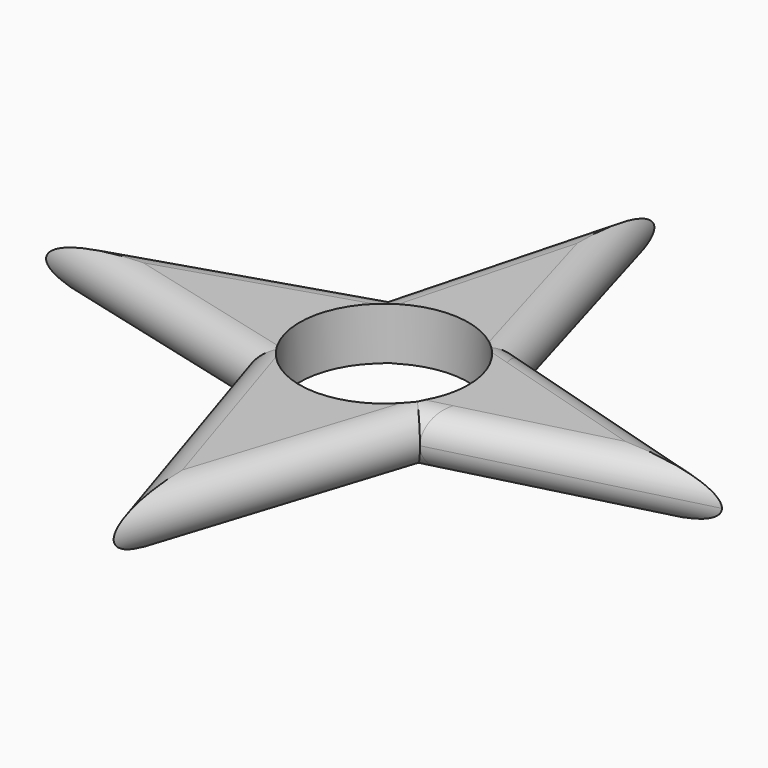
from build123d import *

# Parameters (mm, degrees)
F0_R         = 11.25
F1_DEPTH     = 7
F2_T4_DEPTH  = 53.5102509631
F2_T9_DEPTH  = 52.2381371755
F2_T14_DEPTH = 55.3419579342
F2_T19_DEPTH = 51.9229754131
F2_T24_DEPTH = 55.7195375849
F2_T29_DEPTH = 55.7195375849
F2_T34_DEPTH = 51.9229754131
F2_T39_DEPTH = 53.9484048993
F2_T45_DEPTH = 53.9484048993
F2_T49_DEPTH = 53.5102509631
F2_T56_DEPTH = 52.2381371755
F2_T60_DEPTH = 55.3419579342
F2_T67_DEPTH = 55.7195375849
F2_T71_DEPTH = 51.9229754131
F2_T78_DEPTH = 55.7195375849
F2_T82_DEPTH = 51.9229754131
F3_T4_DEPTH  = 53.5102509631
F3_T9_DEPTH  = 53.9484048993
F3_T14_DEPTH = 51.9229754131
F3_T19_DEPTH = 55.7195375849
F3_T24_DEPTH = 55.7195375849
F3_T29_DEPTH = 51.9229754131
F3_T34_DEPTH = 55.3419579342
F3_T39_DEPTH = 52.2381371755
F3_T45_DEPTH = 53.5102509631
F3_T49_DEPTH = 53.9484048993
F3_T56_DEPTH = 51.9229754131
F3_T60_DEPTH = 55.7195375849
F3_T67_DEPTH = 55.7195375849
F3_T71_DEPTH = 51.9229754131
F3_T78_DEPTH = 55.3419579342
F3_T82_DEPTH = 52.2381371755


# Not quite as in the source:
# - a fillet or chamfer that OpenCascade refuses, or shapes differently, is made with other operations: its cross-section is extruded or revolved along the edge and cut away or added


with BuildPart() as f1:
    # F0 (on Top) → F1 (new body)
    with BuildSketch(Plane.XY):
        with BuildLine():
            ThreePointArc((11.6700973746, -8.6057438533), (13.7743677156, -4.5295467802), (14.5, 0))
            ThreePointArc((14.5, 0), (13.3480283218, 5.6639332553), (10.0751531144, 10.4279091731))
            ThreePointArc((10.0751531144, 10.4279091731), (0.7621030803, 14.4799585253), (-8.9248468856, 11.4279091731))
            ThreePointArc((-8.9248468856, 11.4279091731), (-14.3657490464, 1.9685665686), (-11.6700973746, -8.6057438533))
            ThreePointArc((-11.6700973746, -8.6057438533), (0, -14.5), (11.6700973746, -8.6057438533))
        make_face()
        Circle(F0_R, mode=Mode.SUBTRACT)
        with BuildLine():
            ThreePointArc((10.0751531144, 10.4279091731), (13.3480283218, 5.6639332553), (14.5, 0))
            ThreePointArc((14.5, 0), (13.7743677156, -4.5295467802), (11.6700973746, -8.6057438533))
            Line((11.6700973746, -8.6057438533), (45, 0))
            Line((45, 0), (10.0751531144, 10.4279091731))
        make_face()
        with BuildLine():
            ThreePointArc((-8.9248468856, 11.4279091731), (0.7621030803, 14.4799585253), (10.0751531144, 10.4279091731))
            Line((10.0751531144, 10.4279091731), (0, 45))
            Line((0, 45), (-8.9248468856, 11.4279091731))
        make_face()
        with BuildLine():
            Line((0, -45), (11.6700973746, -8.6057438533))
            ThreePointArc((11.6700973746, -8.6057438533), (0, -14.5), (-11.6700973746, -8.6057438533))
            Line((-11.6700973746, -8.6057438533), (0, -45))
        make_face()
        with BuildLine():
            ThreePointArc((-11.6700973746, -8.6057438533), (-14.3657490464, 1.9685665686), (-8.9248468856, 11.4279091731))
            Line((-8.9248468856, 11.4279091731), (-45, 0))
            Line((-45, 0), (-11.6700973746, -8.6057438533))
        make_face()
    extrude(amount=F1_DEPTH)

    # F2: fillet of radius 3.5 on 8 edges, made by hand


with BuildPart() as f2_tool2:
    # F2_s3 → F2_t4 (new body)
    with BuildSketch(Plane(origin=(0.4357492619, -1.4952391183, 0), x_dir=(0, 0, 1), z_dir=(-0.2797856956, 0.9600624795, 0))):
        with BuildLine():
            ThreePointArc((3.5, 12.5903563019), (5.9748737342, 11.5652300361), (7, 9.0903563019))
            Line((7, 9.0903563019), (7, 12.5903563019))
            Line((7, 12.5903563019), (3.5, 12.5903563019))
        make_face()
    extrude(amount=F2_T4_DEPTH)

    split(bisect_by=Plane(origin=(3.6834089544, 12.3363650004, 0), x_dir=(0, 0, 1), z_dir=(0.2861005633, 0.958199597, 0)), keep=Keep.TOP)


with BuildPart() as f1_1:
    add(f1.part)

    # F2_t1: cut F2_tool2
    add(f2_tool2.part, mode=Mode.SUBTRACT)


with BuildPart() as f2_tool7:
    # F2_s8 → F2_t9 (new body)
    with BuildSketch(Plane(origin=(13.4212581193, 50.4859861874, 0), x_dir=(0, 0, 1), z_dir=(-0.2569178318, -0.9664332505, 0))):
        with BuildLine():
            ThreePointArc((3.5, 11.5613024332), (5.9748737342, 10.5361761674), (7, 8.0613024332))
            Line((7, 8.0613024332), (7, 11.5613024332))
            Line((7, 11.5613024332), (3.5, 11.5613024332))
        make_face()
    extrude(amount=F2_T9_DEPTH)

    split(bisect_by=Plane(origin=(-4.1039199091, 12.9550853833, 0), x_dir=(0, 0, 1), z_dir=(-0.3019904306, 0.9533109565, 0)), keep=Keep.TOP)


with BuildPart() as f1_2:
    add(f1_1.part)

    # F2_t6: cut F2_tool7
    add(f2_tool7.part, mode=Mode.SUBTRACT)


with BuildPart() as f2_tool12:
    # F2_s13 → F2_t14 (new body)
    with BuildSketch(Plane(origin=(3.5205438929, 1.1152400579, 0), x_dir=(0, 0, 1), z_dir=(-0.9533109565, -0.3019904306, 0))):
        with BuildLine():
            ThreePointArc((3.5, 13.5895693791), (5.9748737342, 12.5644431133), (7, 10.0895693791))
            Line((7, 10.0895693791), (7, 13.5895693791))
            Line((7, 13.5895693791), (3.5, 13.5895693791))
        make_face()
    extrude(amount=F2_T14_DEPTH)

    split(bisect_by=Plane(origin=(-11.1732270906, 2.9703047545, 0), x_dir=(0, 0, 1), z_dir=(-0.9664332505, 0.2569178318, 0)), keep=Keep.TOP)


with BuildPart() as f1_3:
    add(f1_2.part)

    # F2_t11: cut F2_tool12
    add(f2_tool12.part, mode=Mode.SUBTRACT)


with BuildPart() as f2_tool17:
    # F2_s18 → F2_t19 (new body)
    with BuildSketch(Plane(origin=(-50.6596510698, 13.0802656612, 0), x_dir=(0, 0, 1), z_dir=(0.9682458366, -0.25, 0))):
        with BuildLine():
            ThreePointArc((3.5, 11.25), (5.9748737342, 10.2248737342), (7, 7.75))
            Line((7, 7.75), (7, 11.25))
            Line((7, 11.25), (3.5, 11.25))
        make_face()
    extrude(amount=F2_T19_DEPTH)

    split(bisect_by=Plane(origin=(-13.0842545446, -4.1955665749, 0), x_dir=(0, 0, 1), z_dir=(-0.9522421894, -0.3053437616, 0)), keep=Keep.TOP)


with BuildPart() as f1_4:
    add(f1_3.part)

    # F2_t16: cut F2_tool17
    add(f2_tool17.part, mode=Mode.SUBTRACT)


with BuildPart() as f2_tool22:
    # F2_s23 → F2_t24 (new body)
    with BuildSketch(Plane(origin=(-1.2576007444, 3.9219418787, 0), x_dir=(0, 0, 1), z_dir=(0.3053437616, -0.9522421894, 0))):
        with BuildLine():
            ThreePointArc((3.5, 13.7404692741), (5.9748737342, 12.7153430082), (7, 10.2404692741))
            Line((7, 10.2404692741), (7, 13.7404692741))
            Line((7, 13.7404692741), (3.5, 13.7404692741))
        make_face()
    extrude(amount=F2_T24_DEPTH)

    split(bisect_by=Plane(origin=(-2.8125, -10.8927656612, 0), x_dir=(0, 0, 1), z_dir=(-0.25, -0.9682458366, 0)), keep=Keep.TOP)


with BuildPart() as f1_5:
    add(f1_4.part)

    # F2_t21: cut F2_tool22
    add(f2_tool22.part, mode=Mode.SUBTRACT)


with BuildPart() as f2_tool27:
    # F2_s28 → F2_t29 (new body)
    with BuildSketch(Plane(origin=(-15.756012459, -49.1365525821, 0), x_dir=(0, 0, 1), z_dir=(0.3053437616, 0.9522421894, 0))):
        with BuildLine():
            ThreePointArc((3.5, 13.7404692741), (5.9748737342, 12.7153430082), (7, 10.2404692741))
            Line((7, 10.2404692741), (7, 13.7404692741))
            Line((7, 13.7404692741), (3.5, 13.7404692741))
        make_face()
    extrude(amount=F2_T29_DEPTH)

    split(bisect_by=Plane(origin=(2.8125, -10.8927656612, 0), x_dir=(0, 0, 1), z_dir=(0.25, -0.9682458366, 0)), keep=Keep.TOP)


with BuildPart() as f1_6:
    add(f1_5.part)

    # F2_t26: cut F2_tool27
    add(f2_tool27.part, mode=Mode.SUBTRACT)


with BuildPart() as f2_tool32:
    # F2_s33 → F2_t34 (new body)
    with BuildSketch(Plane(origin=(0.3854463047, 0.0995218079, 0), x_dir=(0, 0, 1), z_dir=(0.9682458366, 0.25, 0))):
        with BuildLine():
            ThreePointArc((3.5, 11.25), (5.9748737342, 10.2248737342), (7, 7.75))
            Line((7, 7.75), (7, 11.25))
            Line((7, 11.25), (3.5, 11.25))
        make_face()
    extrude(amount=F2_T34_DEPTH)

    split(bisect_by=Plane(origin=(13.0842545446, -4.1955665749, 0), x_dir=(0, 0, 1), z_dir=(0.9522421894, -0.3053437616, 0)), keep=Keep.TOP)


with BuildPart() as f1_7:
    add(f1_6.part)

    # F2_t31: cut F2_tool32
    add(f2_tool32.part, mode=Mode.SUBTRACT)


with BuildPart() as f2_tool37:
    # F2_s38 → F2_t39 (new body)
    with BuildSketch(Plane(origin=(49.7008375193, -14.8397449293, 0), x_dir=(0, 0, 1), z_dir=(-0.958199597, 0.2861005633, 0))):
        with BuildLine():
            ThreePointArc((3.5, 12.8745253485), (5.9748737342, 11.8493990826), (7, 9.3745253485))
            Line((7, 9.3745253485), (7, 12.8745253485))
            Line((7, 12.8745253485), (3.5, 12.8745253485))
        make_face()
    extrude(amount=F2_T39_DEPTH)

    split(bisect_by=Plane(origin=(12.087528689, 3.5226015958, 0), x_dir=(0, 0, 1), z_dir=(0.9600624795, 0.2797856956, 0)), keep=Keep.TOP)


with BuildPart() as f1_8:
    add(f1_7.part)

    # F2_t36: cut F2_tool37
    add(f2_tool37.part, mode=Mode.SUBTRACT)


with BuildPart() as f2_tool43:
    # F2_s44 → F2_t45 (new body)
    with BuildSketch(Plane(origin=(49.7008375193, -14.8397449293, 0), x_dir=(0, 0, 1), z_dir=(-0.958199597, 0.2861005633, 0))):
        with BuildLine():
            ThreePointArc((3.5, 12.8745253485), (5.9748737342, 11.8493990826), (7, 9.3745253485))
            Line((7, 9.3745253485), (7, 12.8745253485))
            Line((7, 12.8745253485), (3.5, 12.8745253485))
        make_face()
    extrude(amount=F2_T45_DEPTH)

    split(bisect_by=Plane(origin=(12.087528689, 3.5226015958, 0), x_dir=(0, 0, 1), z_dir=(-0.9600624795, -0.2797856956, 0)), keep=Keep.TOP)


with BuildPart() as f2_tool47:
    # F2_s48 → F2_t49 (new body)
    with BuildSketch(Plane(origin=(0.4357492619, -1.4952391183, 0), x_dir=(0, 0, 1), z_dir=(-0.2797856956, 0.9600624795, 0))):
        with BuildLine():
            ThreePointArc((3.5, 12.5903563019), (5.9748737342, 11.5652300361), (7, 9.0903563019))
            Line((7, 9.0903563019), (7, 12.5903563019))
            Line((7, 12.5903563019), (3.5, 12.5903563019))
        make_face()
    extrude(amount=F2_T49_DEPTH)

    split(bisect_by=Plane(origin=(3.6834089544, 12.3363650004, 0), x_dir=(0, 0, 1), z_dir=(-0.2861005633, -0.958199597, 0)), keep=Keep.TOP)


with BuildPart() as f2_tool43_1:
    add(f2_tool43.part)

    # F2_t51: intersect F2_tool47
    add(f2_tool47.part, mode=Mode.INTERSECT)


with BuildPart() as f1_9:
    add(f1_8.part)

    # F2_t41: cut F2_tool43
    add(f2_tool43_1.part, mode=Mode.SUBTRACT)


with BuildPart() as f2_tool54:
    # F2_s55 → F2_t56 (new body)
    with BuildSketch(Plane(origin=(13.4212581193, 50.4859861874, 0), x_dir=(0, 0, 1), z_dir=(-0.2569178318, -0.9664332505, 0))):
        with BuildLine():
            ThreePointArc((3.5, 11.5613024332), (5.9748737342, 10.5361761674), (7, 8.0613024332))
            Line((7, 8.0613024332), (7, 11.5613024332))
            Line((7, 11.5613024332), (3.5, 11.5613024332))
        make_face()
    extrude(amount=F2_T56_DEPTH)

    split(bisect_by=Plane(origin=(-4.1039199091, 12.9550853833, 0), x_dir=(0, 0, 1), z_dir=(0.3019904306, -0.9533109565, 0)), keep=Keep.TOP)


with BuildPart() as f2_tool58:
    # F2_s59 → F2_t60 (new body)
    with BuildSketch(Plane(origin=(3.5205438929, 1.1152400579, 0), x_dir=(0, 0, 1), z_dir=(-0.9533109565, -0.3019904306, 0))):
        with BuildLine():
            ThreePointArc((3.5, 13.5895693791), (5.9748737342, 12.5644431133), (7, 10.0895693791))
            Line((7, 10.0895693791), (7, 13.5895693791))
            Line((7, 13.5895693791), (3.5, 13.5895693791))
        make_face()
    extrude(amount=F2_T60_DEPTH)

    split(bisect_by=Plane(origin=(-11.1732270906, 2.9703047545, 0), x_dir=(0, 0, 1), z_dir=(0.9664332505, -0.2569178318, 0)), keep=Keep.TOP)


with BuildPart() as f2_tool54_1:
    add(f2_tool54.part)

    # F2_t62: intersect F2_tool58
    add(f2_tool58.part, mode=Mode.INTERSECT)


with BuildPart() as f1_10:
    add(f1_9.part)

    # F2_t52: cut F2_tool54
    add(f2_tool54_1.part, mode=Mode.SUBTRACT)


with BuildPart() as f2_tool65:
    # F2_s66 → F2_t67 (new body)
    with BuildSketch(Plane(origin=(-1.2576007444, 3.9219418787, 0), x_dir=(0, 0, 1), z_dir=(0.3053437616, -0.9522421894, 0))):
        with BuildLine():
            ThreePointArc((3.5, 13.7404692741), (5.9748737342, 12.7153430082), (7, 10.2404692741))
            Line((7, 10.2404692741), (7, 13.7404692741))
            Line((7, 13.7404692741), (3.5, 13.7404692741))
        make_face()
    extrude(amount=F2_T67_DEPTH)

    split(bisect_by=Plane(origin=(-2.8125, -10.8927656612, 0), x_dir=(0, 0, 1), z_dir=(0.25, 0.9682458366, 0)), keep=Keep.TOP)


with BuildPart() as f2_tool69:
    # F2_s70 → F2_t71 (new body)
    with BuildSketch(Plane(origin=(-50.6596510698, 13.0802656612, 0), x_dir=(0, 0, 1), z_dir=(0.9682458366, -0.25, 0))):
        with BuildLine():
            ThreePointArc((3.5, 11.25), (5.9748737342, 10.2248737342), (7, 7.75))
            Line((7, 7.75), (7, 11.25))
            Line((7, 11.25), (3.5, 11.25))
        make_face()
    extrude(amount=F2_T71_DEPTH)

    split(bisect_by=Plane(origin=(-13.0842545446, -4.1955665749, 0), x_dir=(0, 0, 1), z_dir=(0.9522421894, 0.3053437616, 0)), keep=Keep.TOP)


with BuildPart() as f2_tool65_1:
    add(f2_tool65.part)

    # F2_t73: intersect F2_tool69
    add(f2_tool69.part, mode=Mode.INTERSECT)


with BuildPart() as f1_11:
    add(f1_10.part)

    # F2_t63: cut F2_tool65
    add(f2_tool65_1.part, mode=Mode.SUBTRACT)


with BuildPart() as f2_tool76:
    # F2_s77 → F2_t78 (new body)
    with BuildSketch(Plane(origin=(-15.756012459, -49.1365525821, 0), x_dir=(0, 0, 1), z_dir=(0.3053437616, 0.9522421894, 0))):
        with BuildLine():
            ThreePointArc((3.5, 13.7404692741), (5.9748737342, 12.7153430082), (7, 10.2404692741))
            Line((7, 10.2404692741), (7, 13.7404692741))
            Line((7, 13.7404692741), (3.5, 13.7404692741))
        make_face()
    extrude(amount=F2_T78_DEPTH)

    split(bisect_by=Plane(origin=(2.8125, -10.8927656612, 0), x_dir=(0, 0, 1), z_dir=(-0.25, 0.9682458366, 0)), keep=Keep.TOP)


with BuildPart() as f2_tool80:
    # F2_s81 → F2_t82 (new body)
    with BuildSketch(Plane(origin=(0.3854463047, 0.0995218079, 0), x_dir=(0, 0, 1), z_dir=(0.9682458366, 0.25, 0))):
        with BuildLine():
            ThreePointArc((3.5, 11.25), (5.9748737342, 10.2248737342), (7, 7.75))
            Line((7, 7.75), (7, 11.25))
            Line((7, 11.25), (3.5, 11.25))
        make_face()
    extrude(amount=F2_T82_DEPTH)

    split(bisect_by=Plane(origin=(13.0842545446, -4.1955665749, 0), x_dir=(0, 0, 1), z_dir=(-0.9522421894, 0.3053437616, 0)), keep=Keep.TOP)


with BuildPart() as f2_tool76_1:
    add(f2_tool76.part)

    # F2_t84: intersect F2_tool80
    add(f2_tool80.part, mode=Mode.INTERSECT)


with BuildPart() as f1_12:
    add(f1_11.part)

    # F2_t74: cut F2_tool76
    add(f2_tool76_1.part, mode=Mode.SUBTRACT)

    # F3: fillet of radius 3.5 on 8 edges, made by hand


with BuildPart() as f3_tool2:
    # F3_s3 → F3_t4 (new body)
    with BuildSketch(Plane(origin=(0.4357492619, -1.4952391183, 0), x_dir=(0, 0, 1), z_dir=(-0.2797856956, 0.9600624795, 0))):
        with BuildLine():
            ThreePointArc((3.5, 12.5903563019), (1.0251262658, 11.5652300361), (0, 9.0903563019))
            Line((0, 9.0903563019), (0, 12.5903563019))
            Line((0, 12.5903563019), (3.5, 12.5903563019))
        make_face()
    extrude(amount=F3_T4_DEPTH)

    split(bisect_by=Plane(origin=(3.6834089544, 12.3363650004, 0), x_dir=(0, 0, 1), z_dir=(0.2861005633, 0.958199597, 0)), keep=Keep.TOP)


with BuildPart() as f1_13:
    add(f1_12.part)

    # F3_t1: cut F3_tool2
    add(f3_tool2.part, mode=Mode.SUBTRACT)


with BuildPart() as f3_tool7:
    # F3_s8 → F3_t9 (new body)
    with BuildSketch(Plane(origin=(49.7008375193, -14.8397449293, 0), x_dir=(0, 0, 1), z_dir=(-0.958199597, 0.2861005633, 0))):
        with BuildLine():
            ThreePointArc((3.5, 12.8745253485), (1.0251262658, 11.8493990826), (0, 9.3745253485))
            Line((0, 9.3745253485), (0, 12.8745253485))
            Line((0, 12.8745253485), (3.5, 12.8745253485))
        make_face()
    extrude(amount=F3_T9_DEPTH)

    split(bisect_by=Plane(origin=(12.087528689, 3.5226015958, 0), x_dir=(0, 0, 1), z_dir=(0.9600624795, 0.2797856956, 0)), keep=Keep.TOP)


with BuildPart() as f1_14:
    add(f1_13.part)

    # F3_t6: cut F3_tool7
    add(f3_tool7.part, mode=Mode.SUBTRACT)


with BuildPart() as f3_tool12:
    # F3_s13 → F3_t14 (new body)
    with BuildSketch(Plane(origin=(0.3854463047, 0.0995218079, 0), x_dir=(0, 0, 1), z_dir=(0.9682458366, 0.25, 0))):
        with BuildLine():
            ThreePointArc((3.5, 11.25), (1.0251262658, 10.2248737342), (0, 7.75))
            Line((0, 7.75), (0, 11.25))
            Line((0, 11.25), (3.5, 11.25))
        make_face()
    extrude(amount=F3_T14_DEPTH)

    split(bisect_by=Plane(origin=(13.0842545446, -4.1955665749, 0), x_dir=(0, 0, 1), z_dir=(0.9522421894, -0.3053437616, 0)), keep=Keep.TOP)


with BuildPart() as f1_15:
    add(f1_14.part)

    # F3_t11: cut F3_tool12
    add(f3_tool12.part, mode=Mode.SUBTRACT)


with BuildPart() as f3_tool17:
    # F3_s18 → F3_t19 (new body)
    with BuildSketch(Plane(origin=(-15.756012459, -49.1365525821, 0), x_dir=(0, 0, 1), z_dir=(0.3053437616, 0.9522421894, 0))):
        with BuildLine():
            ThreePointArc((3.5, 13.7404692741), (1.0251262658, 12.7153430082), (0, 10.2404692741))
            Line((0, 10.2404692741), (0, 13.7404692741))
            Line((0, 13.7404692741), (3.5, 13.7404692741))
        make_face()
    extrude(amount=F3_T19_DEPTH)

    split(bisect_by=Plane(origin=(2.8125, -10.8927656612, 0), x_dir=(0, 0, 1), z_dir=(0.25, -0.9682458366, 0)), keep=Keep.TOP)


with BuildPart() as f1_16:
    add(f1_15.part)

    # F3_t16: cut F3_tool17
    add(f3_tool17.part, mode=Mode.SUBTRACT)


with BuildPart() as f3_tool22:
    # F3_s23 → F3_t24 (new body)
    with BuildSketch(Plane(origin=(-1.2576007444, 3.9219418787, 0), x_dir=(0, 0, 1), z_dir=(0.3053437616, -0.9522421894, 0))):
        with BuildLine():
            ThreePointArc((3.5, 13.7404692741), (1.0251262658, 12.7153430082), (0, 10.2404692741))
            Line((0, 10.2404692741), (0, 13.7404692741))
            Line((0, 13.7404692741), (3.5, 13.7404692741))
        make_face()
    extrude(amount=F3_T24_DEPTH)

    split(bisect_by=Plane(origin=(-2.8125, -10.8927656612, 0), x_dir=(0, 0, 1), z_dir=(-0.25, -0.9682458366, 0)), keep=Keep.TOP)


with BuildPart() as f1_17:
    add(f1_16.part)

    # F3_t21: cut F3_tool22
    add(f3_tool22.part, mode=Mode.SUBTRACT)


with BuildPart() as f3_tool27:
    # F3_s28 → F3_t29 (new body)
    with BuildSketch(Plane(origin=(-50.6596510698, 13.0802656612, 0), x_dir=(0, 0, 1), z_dir=(0.9682458366, -0.25, 0))):
        with BuildLine():
            ThreePointArc((3.5, 11.25), (1.0251262658, 10.2248737342), (0, 7.75))
            Line((0, 7.75), (0, 11.25))
            Line((0, 11.25), (3.5, 11.25))
        make_face()
    extrude(amount=F3_T29_DEPTH)

    split(bisect_by=Plane(origin=(-13.0842545446, -4.1955665749, 0), x_dir=(0, 0, 1), z_dir=(-0.9522421894, -0.3053437616, 0)), keep=Keep.TOP)


with BuildPart() as f1_18:
    add(f1_17.part)

    # F3_t26: cut F3_tool27
    add(f3_tool27.part, mode=Mode.SUBTRACT)


with BuildPart() as f3_tool32:
    # F3_s33 → F3_t34 (new body)
    with BuildSketch(Plane(origin=(3.5205438929, 1.1152400579, 0), x_dir=(0, 0, 1), z_dir=(-0.9533109565, -0.3019904306, 0))):
        with BuildLine():
            ThreePointArc((3.5, 13.5895693791), (1.0251262658, 12.5644431133), (0, 10.0895693791))
            Line((0, 10.0895693791), (0, 13.5895693791))
            Line((0, 13.5895693791), (3.5, 13.5895693791))
        make_face()
    extrude(amount=F3_T34_DEPTH)

    split(bisect_by=Plane(origin=(-11.1732270906, 2.9703047545, 0), x_dir=(0, 0, 1), z_dir=(-0.9664332505, 0.2569178318, 0)), keep=Keep.TOP)


with BuildPart() as f1_19:
    add(f1_18.part)

    # F3_t31: cut F3_tool32
    add(f3_tool32.part, mode=Mode.SUBTRACT)


with BuildPart() as f3_tool37:
    # F3_s38 → F3_t39 (new body)
    with BuildSketch(Plane(origin=(13.4212581193, 50.4859861874, 0), x_dir=(0, 0, 1), z_dir=(-0.2569178318, -0.9664332505, 0))):
        with BuildLine():
            ThreePointArc((3.5, 11.5613024332), (1.0251262658, 10.5361761674), (0, 8.0613024332))
            Line((0, 8.0613024332), (0, 11.5613024332))
            Line((0, 11.5613024332), (3.5, 11.5613024332))
        make_face()
    extrude(amount=F3_T39_DEPTH)

    split(bisect_by=Plane(origin=(-4.1039199091, 12.9550853833, 0), x_dir=(0, 0, 1), z_dir=(-0.3019904306, 0.9533109565, 0)), keep=Keep.TOP)


with BuildPart() as f1_20:
    add(f1_19.part)

    # F3_t36: cut F3_tool37
    add(f3_tool37.part, mode=Mode.SUBTRACT)


with BuildPart() as f3_tool43:
    # F3_s44 → F3_t45 (new body)
    with BuildSketch(Plane(origin=(0.4357492619, -1.4952391183, 0), x_dir=(0, 0, 1), z_dir=(-0.2797856956, 0.9600624795, 0))):
        with BuildLine():
            ThreePointArc((3.5, 12.5903563019), (1.0251262658, 11.5652300361), (0, 9.0903563019))
            Line((0, 9.0903563019), (0, 12.5903563019))
            Line((0, 12.5903563019), (3.5, 12.5903563019))
        make_face()
    extrude(amount=F3_T45_DEPTH)

    split(bisect_by=Plane(origin=(3.6834089544, 12.3363650004, 0), x_dir=(0, 0, 1), z_dir=(-0.2861005633, -0.958199597, 0)), keep=Keep.TOP)


with BuildPart() as f3_tool47:
    # F3_s48 → F3_t49 (new body)
    with BuildSketch(Plane(origin=(49.7008375193, -14.8397449293, 0), x_dir=(0, 0, 1), z_dir=(-0.958199597, 0.2861005633, 0))):
        with BuildLine():
            ThreePointArc((3.5, 12.8745253485), (1.0251262658, 11.8493990826), (0, 9.3745253485))
            Line((0, 9.3745253485), (0, 12.8745253485))
            Line((0, 12.8745253485), (3.5, 12.8745253485))
        make_face()
    extrude(amount=F3_T49_DEPTH)

    split(bisect_by=Plane(origin=(12.087528689, 3.5226015958, 0), x_dir=(0, 0, 1), z_dir=(-0.9600624795, -0.2797856956, 0)), keep=Keep.TOP)


with BuildPart() as f3_tool43_1:
    add(f3_tool43.part)

    # F3_t51: intersect F3_tool47
    add(f3_tool47.part, mode=Mode.INTERSECT)


with BuildPart() as f1_21:
    add(f1_20.part)

    # F3_t41: cut F3_tool43
    add(f3_tool43_1.part, mode=Mode.SUBTRACT)


with BuildPart() as f3_tool54:
    # F3_s55 → F3_t56 (new body)
    with BuildSketch(Plane(origin=(0.3854463047, 0.0995218079, 0), x_dir=(0, 0, 1), z_dir=(0.9682458366, 0.25, 0))):
        with BuildLine():
            ThreePointArc((3.5, 11.25), (1.0251262658, 10.2248737342), (0, 7.75))
            Line((0, 7.75), (0, 11.25))
            Line((0, 11.25), (3.5, 11.25))
        make_face()
    extrude(amount=F3_T56_DEPTH)

    split(bisect_by=Plane(origin=(13.0842545446, -4.1955665749, 0), x_dir=(0, 0, 1), z_dir=(-0.9522421894, 0.3053437616, 0)), keep=Keep.TOP)


with BuildPart() as f3_tool58:
    # F3_s59 → F3_t60 (new body)
    with BuildSketch(Plane(origin=(-15.756012459, -49.1365525821, 0), x_dir=(0, 0, 1), z_dir=(0.3053437616, 0.9522421894, 0))):
        with BuildLine():
            ThreePointArc((3.5, 13.7404692741), (1.0251262658, 12.7153430082), (0, 10.2404692741))
            Line((0, 10.2404692741), (0, 13.7404692741))
            Line((0, 13.7404692741), (3.5, 13.7404692741))
        make_face()
    extrude(amount=F3_T60_DEPTH)

    split(bisect_by=Plane(origin=(2.8125, -10.8927656612, 0), x_dir=(0, 0, 1), z_dir=(-0.25, 0.9682458366, 0)), keep=Keep.TOP)


with BuildPart() as f3_tool54_1:
    add(f3_tool54.part)

    # F3_t62: intersect F3_tool58
    add(f3_tool58.part, mode=Mode.INTERSECT)


with BuildPart() as f1_22:
    add(f1_21.part)

    # F3_t52: cut F3_tool54
    add(f3_tool54_1.part, mode=Mode.SUBTRACT)


with BuildPart() as f3_tool65:
    # F3_s66 → F3_t67 (new body)
    with BuildSketch(Plane(origin=(-1.2576007444, 3.9219418787, 0), x_dir=(0, 0, 1), z_dir=(0.3053437616, -0.9522421894, 0))):
        with BuildLine():
            ThreePointArc((3.5, 13.7404692741), (1.0251262658, 12.7153430082), (0, 10.2404692741))
            Line((0, 10.2404692741), (0, 13.7404692741))
            Line((0, 13.7404692741), (3.5, 13.7404692741))
        make_face()
    extrude(amount=F3_T67_DEPTH)

    split(bisect_by=Plane(origin=(-2.8125, -10.8927656612, 0), x_dir=(0, 0, 1), z_dir=(0.25, 0.9682458366, 0)), keep=Keep.TOP)


with BuildPart() as f3_tool69:
    # F3_s70 → F3_t71 (new body)
    with BuildSketch(Plane(origin=(-50.6596510698, 13.0802656612, 0), x_dir=(0, 0, 1), z_dir=(0.9682458366, -0.25, 0))):
        with BuildLine():
            ThreePointArc((3.5, 11.25), (1.0251262658, 10.2248737342), (0, 7.75))
            Line((0, 7.75), (0, 11.25))
            Line((0, 11.25), (3.5, 11.25))
        make_face()
    extrude(amount=F3_T71_DEPTH)

    split(bisect_by=Plane(origin=(-13.0842545446, -4.1955665749, 0), x_dir=(0, 0, 1), z_dir=(0.9522421894, 0.3053437616, 0)), keep=Keep.TOP)


with BuildPart() as f3_tool65_1:
    add(f3_tool65.part)

    # F3_t73: intersect F3_tool69
    add(f3_tool69.part, mode=Mode.INTERSECT)


with BuildPart() as f1_23:
    add(f1_22.part)

    # F3_t63: cut F3_tool65
    add(f3_tool65_1.part, mode=Mode.SUBTRACT)


with BuildPart() as f3_tool76:
    # F3_s77 → F3_t78 (new body)
    with BuildSketch(Plane(origin=(3.5205438929, 1.1152400579, 0), x_dir=(0, 0, 1), z_dir=(-0.9533109565, -0.3019904306, 0))):
        with BuildLine():
            ThreePointArc((3.5, 13.5895693791), (1.0251262658, 12.5644431133), (0, 10.0895693791))
            Line((0, 10.0895693791), (0, 13.5895693791))
            Line((0, 13.5895693791), (3.5, 13.5895693791))
        make_face()
    extrude(amount=F3_T78_DEPTH)

    split(bisect_by=Plane(origin=(-11.1732270906, 2.9703047545, 0), x_dir=(0, 0, 1), z_dir=(0.9664332505, -0.2569178318, 0)), keep=Keep.TOP)


with BuildPart() as f3_tool80:
    # F3_s81 → F3_t82 (new body)
    with BuildSketch(Plane(origin=(13.4212581193, 50.4859861874, 0), x_dir=(0, 0, 1), z_dir=(-0.2569178318, -0.9664332505, 0))):
        with BuildLine():
            ThreePointArc((3.5, 11.5613024332), (1.0251262658, 10.5361761674), (0, 8.0613024332))
            Line((0, 8.0613024332), (0, 11.5613024332))
            Line((0, 11.5613024332), (3.5, 11.5613024332))
        make_face()
    extrude(amount=F3_T82_DEPTH)

    split(bisect_by=Plane(origin=(-4.1039199091, 12.9550853833, 0), x_dir=(0, 0, 1), z_dir=(0.3019904306, -0.9533109565, 0)), keep=Keep.TOP)


with BuildPart() as f3_tool76_1:
    add(f3_tool76.part)

    # F3_t84: intersect F3_tool80
    add(f3_tool80.part, mode=Mode.INTERSECT)


with BuildPart() as f1_24:
    add(f1_23.part)

    # F3_t74: cut F3_tool76
    add(f3_tool76_1.part, mode=Mode.SUBTRACT)


solid = f1_24.part
